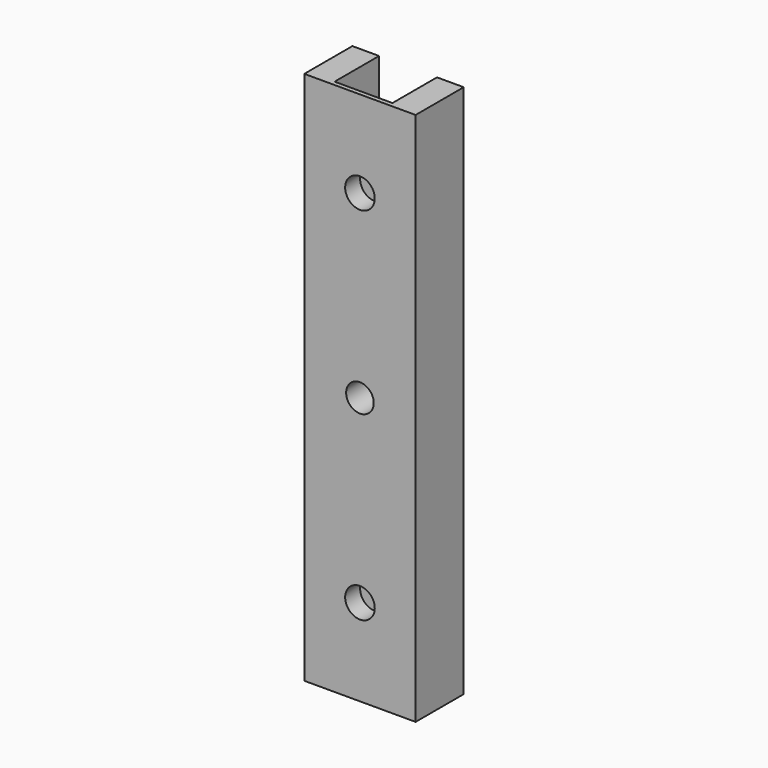
from build123d import *

# Parameters (mm, degrees)
F0_W        = 25
F0_H        = 120
F1_DEPTH    = 13.5
F2_R        = 3.1
F3_DEPTH    = 13.501
F4_W        = 13
F4_H        = 17.8598619506
F5_DEPTH    = 12.5
F6_R        = 3.325
F7_DEPTH    = 4.2
F8_T        = 3.5
F8_T3_DEPTH = 19.5
F8_T5_DEPTH = 23
F8_T7_DEPTH = 20
F8_T9_DEPTH = 23


# Not quite as in the source:
# - a shell that OpenCascade refuses in one call is made with other operations: the cavity is built on its own and cut out


with BuildPart() as f1:
    # F0 (on Front) → F1 (new body)
    with BuildSketch(Plane.XZ):
        Rectangle(F0_W, F0_H)
    extrude(amount=F1_DEPTH)

    # F2 (on face) → F3 (cut, through all)
    with BuildSketch(Plane.XZ.offset(13.5)):
        Circle(F2_R)
    extrude(amount=-F3_DEPTH, mode=Mode.SUBTRACT)

    # F4 (on face) → F5 (cut)
    with BuildSketch(Plane(origin=(0, 0, 0), x_dir=(-1, 0, 0), z_dir=(0, 1, 0))):
        with Locations((0, 52.9299309753)):
            Rectangle(F4_W, F4_H)
        with Locations((0, -52.9299309753)):
            Rectangle(F4_W, F4_H)
    extrude(amount=-F5_DEPTH, mode=Mode.SUBTRACT)

    # F6 (on face) → F7 (cut)
    with BuildSketch(Plane.XZ.offset(13.5)):
        with Locations((0, -40.5)):
            Circle(F6_R)
        with Locations((0, 40.5)):
            Circle(F6_R)
    extrude(amount=-F7_DEPTH, mode=Mode.SUBTRACT)

    # F8: shell of thickness 3.5, made by hand


with BuildPart() as f8_core1:
    # F8_t2: copy of F1
    add(f1.part)

    # the walls: a layer under each face that stays
    f8_faces = [f8_core1.faces().sort_by_distance(p)[0] for p in [
        (12.5, -6.75, 0),
        (-8.3333333333, -11.25, -60),
        (8.3333333333, -11.25, 60),
        (-8.3333333333, -13.5, -40),
        (-6.5, -6.25, -52),
        (0, -12.5, -52),
        (6.5, -6.25, -52),
        (-12.5, -6.75, 0),
        (6.5, -6.25, 52),
        (0, -12.5, 52),
        (-6.5, -6.25, 52),
        (0, -6.25, -44),
        (0, -6.25, 44),
        (-3.1, -6.75, 0),
        (-3.325, -11.4, -40.5),
        (-3.325, -11.4, 40.5),
        (0, -9.3, -40.5),
        (0, -9.3, 40.5),
    ]]
    thicken(f8_faces, amount=-F8_T, mode=Mode.SUBTRACT)

    # F8_s4 → F8_t3 (cut)
    with BuildSketch(Plane.XZ.offset(-3.5)):
        Polygon((-6.465, -44.035), (-10, -44), (-10, -40.5), (-6.5, -40.5), align=None)
        Polygon((6.465, -44.035), (10, -44), (10, -40.5), (6.5, -40.5), align=None)
        Polygon((6.465, 44.035), (10, 44), (10, 40.5), (6.5, 40.5), align=None)
        Polygon((-6.465, 44.035), (-10, 44), (-10, 40.5), (-6.5, 40.5), align=None)
    extrude(amount=F8_T3_DEPTH, mode=Mode.SUBTRACT)

    # F8_s6 → F8_t5 (cut)
    with BuildSketch(Plane.XY.offset(-63.5)):
        Polygon((-6.465, -12.465), (-10, -12.5), (-10, -16), (-6.5, -16), align=None)
        Polygon((6.465, -12.465), (6.5, -16), (10, -16), (10, -12.5), align=None)
    extrude(amount=F8_T5_DEPTH, mode=Mode.SUBTRACT)

    # F8_s8 → F8_t7 (cut)
    with BuildSketch(Plane.YZ.offset(-10)):
        Polygon((-12.465, -44.035), (-16, -44), (-16, -40.5), (-12.5, -40.5), align=None)
        Polygon((-12.465, 44.035), (-16, 44), (-16, 40.5), (-12.5, 40.5), align=None)
    extrude(amount=F8_T7_DEPTH, mode=Mode.SUBTRACT)

    # F8_s10 → F8_t9 (cut)
    with BuildSketch(Plane.XY.offset(40.5)):
        Polygon((6.465, -12.465), (10, -12.5), (10, -16), (6.5, -16), align=None)
        Polygon((-6.465, -12.465), (-6.5, -16), (-10, -16), (-10, -12.5), align=None)
    extrude(amount=F8_T9_DEPTH, mode=Mode.SUBTRACT)

    # F8_s11 → F8_t12 (revolve, cut)
    with BuildSketch(Plane.XY.offset(-40.5)):
        Polygon((3.29, -9.335), (6.825, -9.3), (6.825, -5.8), (3.325, -5.8), align=None)
    revolve(axis=Axis((0, -9.3, -40.5), (0, -1, 0)), mode=Mode.SUBTRACT)

    # F8_s13 → F8_t14 (revolve, cut)
    with BuildSketch(Plane.XY.offset(40.5)):
        Polygon((3.29, -9.335), (6.825, -9.3), (6.825, -5.8), (3.325, -5.8), align=None)
    revolve(axis=Axis((0, -9.3, 40.5), (0, -1, 0)), mode=Mode.SUBTRACT)


with BuildPart() as f1_1:
    add(f1.part)

    # what is left inside the walls is the cavity
    f8_cavity = [f8_core1.part.solids().sort_by_distance(p)[0] for p in [
        (0, -0.035, -13.5),
    ]]
    add(f8_cavity, mode=Mode.SUBTRACT)


solid = f1_1.part
